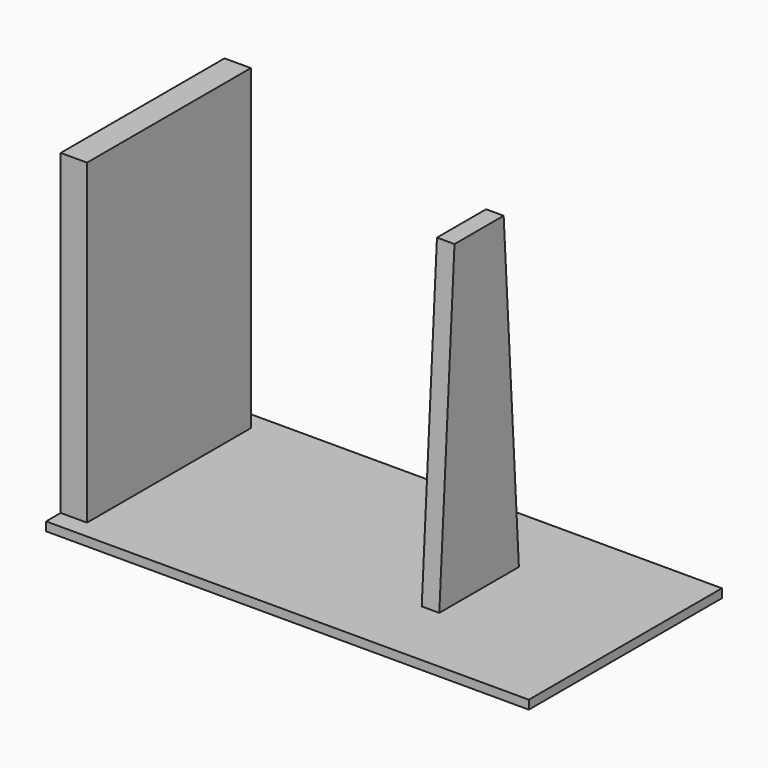
from build123d import *

# Parameters (mm, degrees)
F0_W     = 990
F0_H     = 495
F1_DEPTH = 18
F2_W     = 54
F2_H     = 420
F3_DEPTH = 650
F2_W_2   = 36
F2_H_2   = 204
F4_W     = 204
F4_H     = 650
F5_DEPTH = 690.001
F7_DEPTH = 650
F9_DEPTH = 40


# Not quite as in the source:
# - a feature names something its author has since deleted; it is built from what else it names


with BuildPart() as f1:
    # F0 (on Top) → F1 (new body)
    with BuildSketch(Plane.XY):
        Rectangle(F0_W, F0_H)
    extrude(amount=F1_DEPTH)


with BuildPart() as f3:
    # F2 (on face) → F3 (new body)
    with BuildSketch(Plane.XY.offset(18)):
        with Locations((-468, 0)):
            Rectangle(F2_W, F2_H)
    extrude(amount=F3_DEPTH)


with BuildPart() as f3b:
    # F2 (on face) → F3, piece 2 (new body)
    with BuildSketch(Plane.XY.offset(18)):
        with Locations((177, 0)):
            Rectangle(F2_W_2, F2_H_2)
    extrude(amount=F3_DEPTH)


with BuildPart() as f5_tool:
    # F4 (on face) → F5 (new body, through all)
    with BuildSketch(Plane.YZ.offset(195)):
        with Locations((0, 343)):
            Rectangle(F4_W, F4_H)
    extrude(amount=-F5_DEPTH)


with BuildPart() as f3_1:
    add(f3.part)

    # F5: cut by f5_tool
    add(f5_tool.part, mode=Mode.SUBTRACT)

    # F2 (on face) → F7 (join)
    with BuildSketch(Plane.XY.offset(18)):
        with Locations((-468, 0)):
            Rectangle(F2_W, F2_H)
    extrude(amount=F7_DEPTH)


with BuildPart() as f3b_1:
    add(f3b.part)

    # F5: cut by f5_tool
    add(f5_tool.part, mode=Mode.SUBTRACT)


with BuildPart() as f7:
    # F2 (on face) → F7, piece 2 (new body)
    with BuildSketch(Plane.XY.offset(18)):
        with Locations((177, 0)):
            Rectangle(F2_W_2, F2_H_2)
    extrude(amount=F7_DEPTH)

    # F8 (on face) → F9 (cut)
    with BuildSketch(Plane.YZ.offset(195)):
        Polygon((102, 668), (63, 668), (102, 18), align=None)
        Polygon((-102, 18), (-63, 668), (-102, 668), align=None)
    extrude(amount=-F9_DEPTH, mode=Mode.SUBTRACT)


solid = Compound([f1.part, f3_1.part, f7.part])
